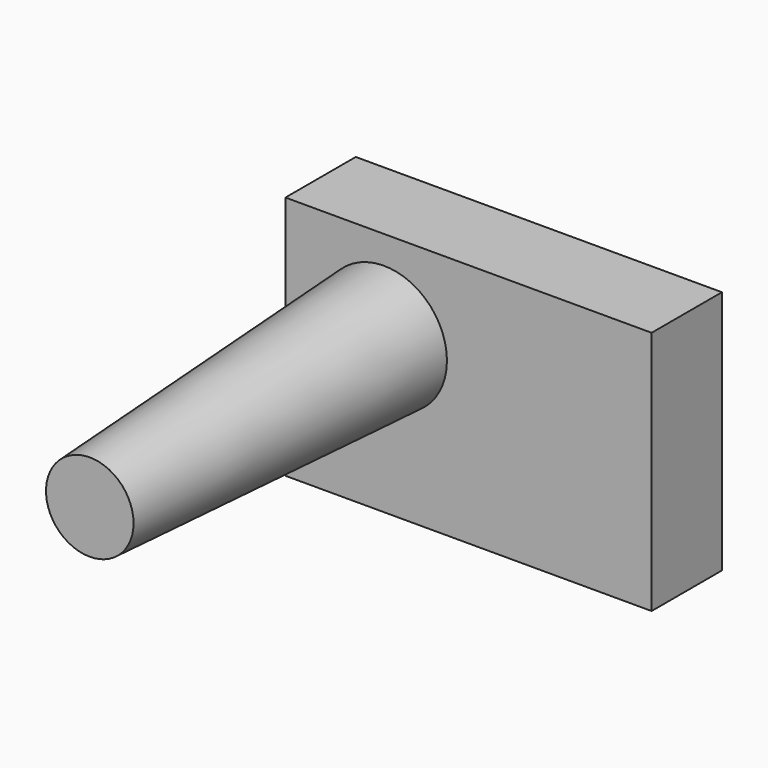
from build123d import *

# Parameters (mm, degrees)
F0_W     = 105.8307476342
F0_H     = 70.8000324667
F1_DEPTH = 25.4
F2_R     = 18.2213910868
F3_DEPTH = 106.25713
F3_TAPER = 3


# Not quite as in the source:
# - the program builds the solid bodies; features that only make, move or delete a surface that nothing else refers to are left out


with BuildPart() as f1:
    # F0 (on Front) → F1 (new body)
    with BuildSketch(Plane.XZ):
        with Locations((-15.6768169254, 19.381063059)):
            Rectangle(F0_W, F0_H)
    extrude(amount=F1_DEPTH)

    # F2 (on face) → F3 (join)
    with BuildSketch(Plane.XZ.offset(25.4)):
        with Locations((-40.1370152831, 28.4684468061)):
            Circle(F2_R)
    extrude(amount=F3_DEPTH, taper=F3_TAPER)


solid = f1.part
